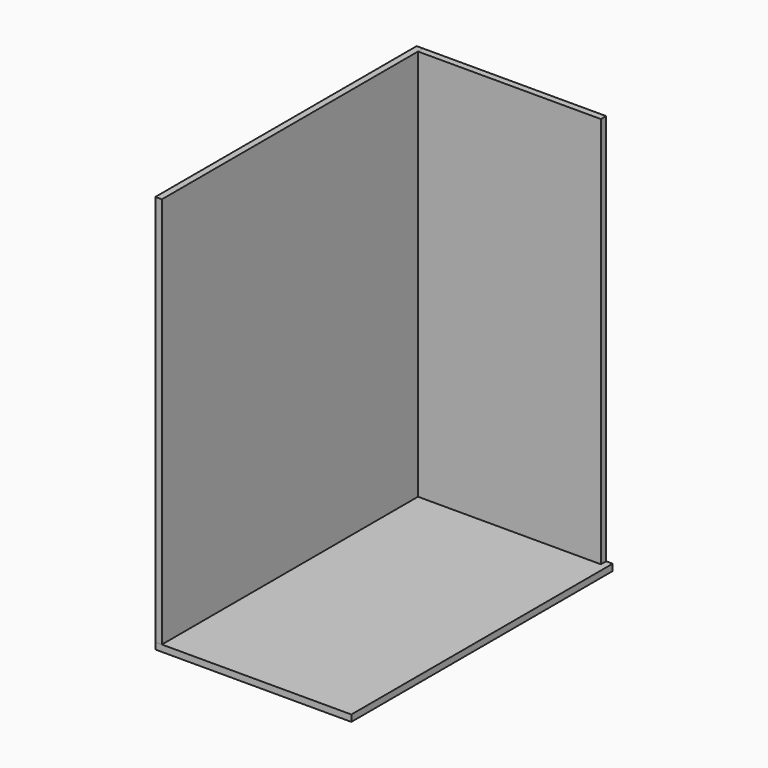
from build123d import *

# Parameters (mm, degrees)
F0_W     = 381
F0_H     = 635
F3_DEPTH = 12.7
F5_DEPTH = 762
F4_W     = 355.6
F4_H     = 12.7
F6_DEPTH = 762


# Not quite as in the source:
# - a variable given as a bare number and used for a length is read in inches; the dataset says mm whatever the document's units were


with BuildPart() as f3:
    # F0 (on Top) → F3 (new body)
    with BuildSketch(Plane.XY):
        Rectangle(F0_W, F0_H)
    extrude(amount=F3_DEPTH)


with BuildPart() as f5:
    # F4 (on face) → F5 (new body)
    with BuildSketch(Plane.XY.offset(12.7)):
        Polygon((-190.5, 317.5), (-190.5, -317.5), (-177.8, -317.5), (-177.8, 304.8), (-177.8, 317.5), align=None)
    extrude(amount=F5_DEPTH)


with BuildPart() as f6:
    # F4 (on face) → F6 (new body)
    with BuildSketch(Plane.XY.offset(12.7)):
        with Locations((0, 311.15)):
            Rectangle(F4_W, F4_H)
    extrude(amount=F6_DEPTH)


solid = Compound([f3.part, f5.part, f6.part])
